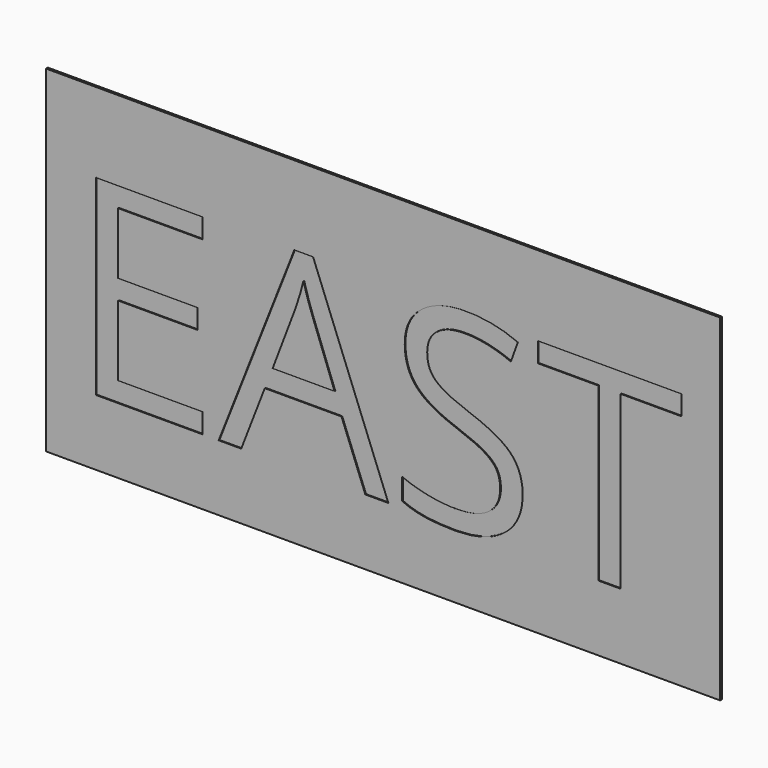
from build123d import *

# Parameters (mm, degrees)
F0_W         = 38.1
F0_H         = 19.05
F1_DEPTH     = 0.127
F2_TEXT_SIZE = 15.1540817685
F3_DEPTH     = 0.0508


# Not quite as in the source:
# - Text() gives the source's letters only with a copy of the font that has no kerning and outlines rounded to 1/6400 em; it was checked with that copy


with BuildPart() as f1:
    # F0 (on Front) → F1 (new body)
    with BuildSketch(Plane.XZ):
        with Locations((19.05, 9.525)):
            Rectangle(F0_W, F0_H)
    extrude(amount=F1_DEPTH)

    # F2 (on face) → F3 (cut)
    with BuildSketch(Plane.XZ.offset(0.127)):
        with Locations((1.3300219062, 3.7257757824)):
            Text('EAST', F2_TEXT_SIZE, font='Open Sans', text_align=(TextAlign.LEFT, TextAlign.BOTTOM))
    extrude(amount=-F3_DEPTH, mode=Mode.SUBTRACT)


solid = f1.part
